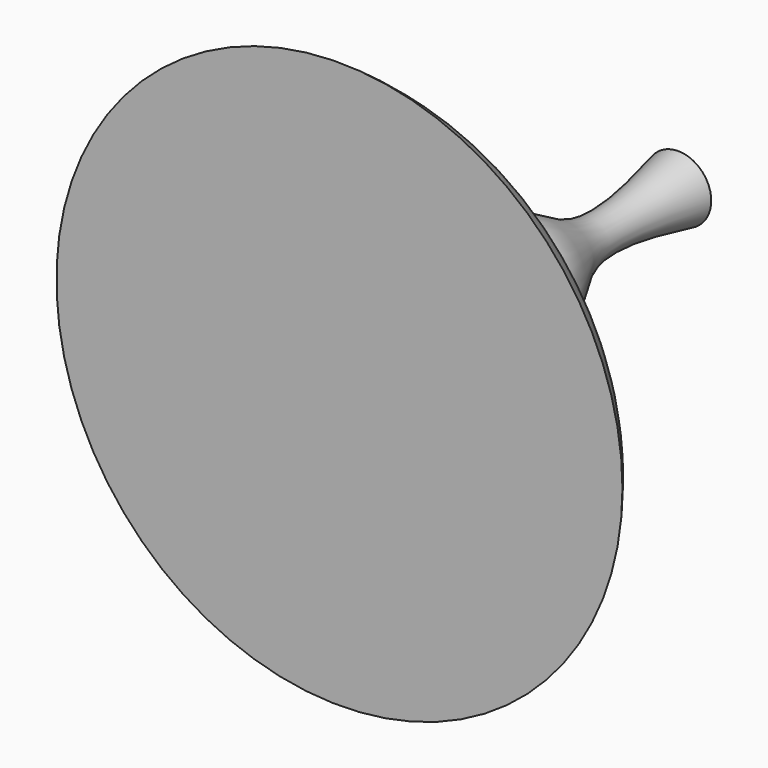
from build123d import *


# Not quite as in the source:
# - a feature of the source that left no trace in its solid (it failed there, or was rolled back) is left out


with BuildPart() as f5:
    # F4 (on Top) → F5 (revolve)
    with BuildSketch(Plane.XY):
        with BuildLine():
            Line((3, 0), (0, 0))
            Line((0, 0), (0, -38.4875983))
            Line((0, -38.4875983), (25.7200915366, -38.4875983))
            add(Edge.make_bspline(
                [(3, 0), (2.0689721237, -4.3065120364), (0.3787112512, -12.1248910313), (7.705129325, -18.3866637047), (-1.5497286946, -32.4215600183), (21.141787172, -32.1481184701), (24.4082681465, -36.6711445957), (25.7200915366, -38.4875983)],
                knots=[0, 0, 0, 0, 0.2113223272, 0.3836510917, 0.5799713529, 0.8313158999, 1, 1, 1, 1], degree=3))
        make_face()
    revolve(axis=Axis((0, -19.24379915, 0), (0, -1, 0)))


solid = f5.part
